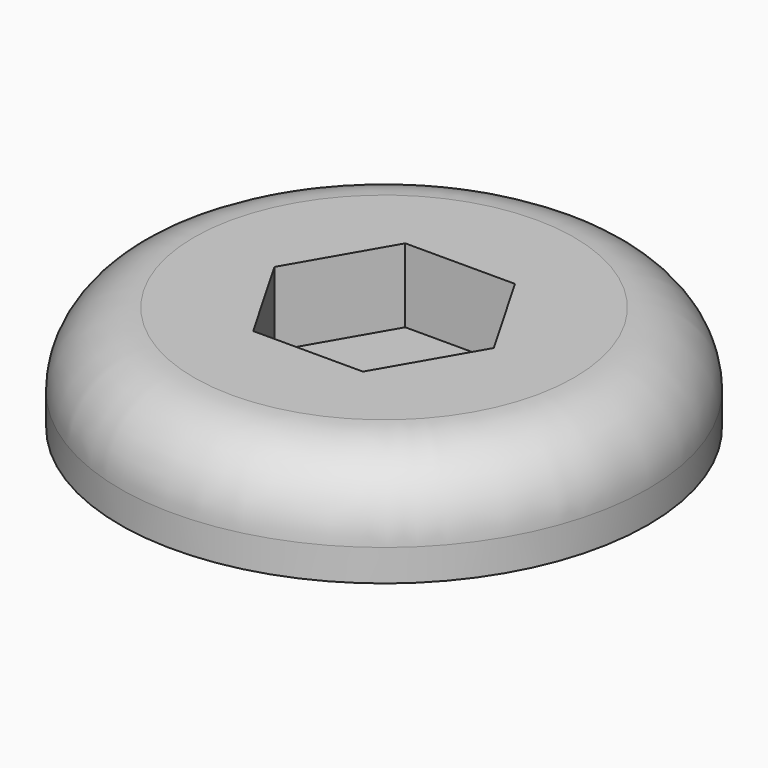
from build123d import *

# Parameters (mm, degrees)
F0_R     = 25
F1_DEPTH = 7
F3_DEPTH = 3
F4_DEPTH = 3
F5_R     = 6.99999


# Not quite as in the source:
# - a fillet or chamfer is up to 0.001 mm smaller than in the source, because OpenCascade refuses the exact size


with BuildPart() as f1:
    # F0 (on Top) → F1 (new body)
    with BuildSketch(Plane.XY):
        Circle(F0_R)
        Polygon((-10.3923048454, 0), (-5.1961524227, 9), (0, 9), (5.1961524227, 9), (10.3923048454, 0), (5.1961524227, -9), (-5.1961524227, -9), align=None, mode=Mode.SUBTRACT)
    extrude(amount=F1_DEPTH)


with BuildPart() as f3:
    # F2 (on face) → F3 (new body)
    with BuildSketch(Plane(origin=(0, 0, 0), x_dir=(1, 0, 0), z_dir=(0, 0, -1))):
        Polygon((5.1961524227, 9), (-5.1961524227, 9), (-10.3923048454, 0), (-5.1961524227, -9), (5.1961524227, -9), (10.3923048454, 0), align=None)
    extrude(amount=F3_DEPTH)


with BuildPart() as f4:
    # F4 (new): a face of the model
    f4_faces = [f1.part.faces().sort_by_distance(p)[0] for p in [
        (-24.2928932188, 0, 0),
    ]]
    extrude(f4_faces, amount=F4_DEPTH)


with BuildPart() as f1_1:
    add(f1.part)

    # F5 (radius 7 in the source; OpenCascade refuses exactly that, so slightly less here)
    f5_edges = [f1_1.edges().sort_by_distance(p)[0] for p in [
        (-25, 0, 7),
    ]]
    fillet(f5_edges, radius=F5_R)


solid = Compound([f3.part, f4.part, f1_1.part])
